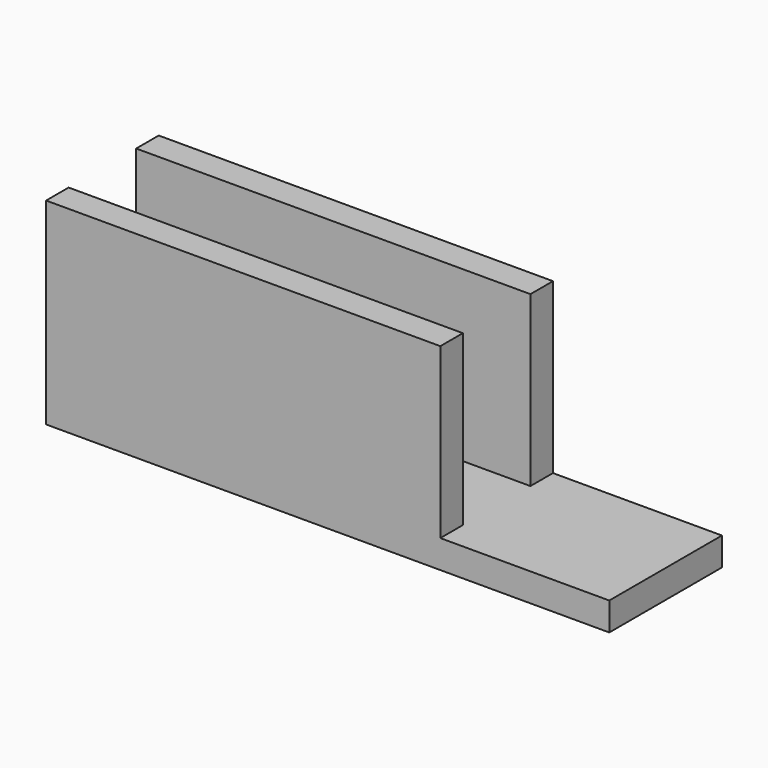
from build123d import *

# Parameters (mm, degrees)
F0_W     = 31.75
F0_H     = 7.9375
F1_DEPTH = 11.1125
F2_W     = 9.525
F2_H     = 7.9375
F3_DEPTH = 9.525
F4_W     = 4.7625
F4_H     = 9.525
F5_DEPTH = 22.226


# Not quite as in the source:
# - a length typed as a fraction of an inch, garbled in the dataset ("3 / 203.2 mm" for 3/8 in), is restored


with BuildPart() as f1:
    # F0 (on Top) → F1 (new body)
    with BuildSketch(Plane.XY):
        with Locations((-0.0819904208, 12.7078423367)):
            Rectangle(F0_W, F0_H)
    extrude(amount=F1_DEPTH)

    # F2 (on face) → F3 (cut)
    with BuildSketch(Plane.XY.offset(11.1125)):
        with Locations((11.0305095792, 12.7078423367)):
            Rectangle(F2_W, F2_H)
    extrude(amount=-F3_DEPTH, mode=Mode.SUBTRACT)

    # F4 (on face) → F5 (cut, through all)
    with BuildSketch(Plane.YZ.offset(6.2680095792)):
        with Locations((12.7078423367, 6.35)):
            Rectangle(F4_W, F4_H)
    extrude(amount=-F5_DEPTH, mode=Mode.SUBTRACT)


solid = f1.part
